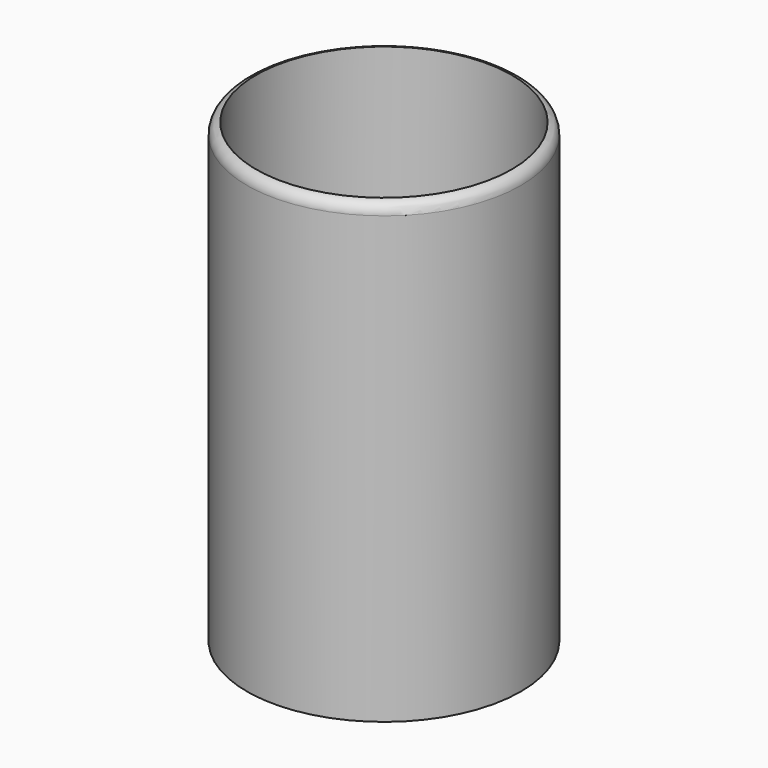
from build123d import *

# Parameters (mm, degrees)
F0_R     = 38.1
F1_DEPTH = 127
F2_T     = -2.54


# Not quite as in the source:
# - a fillet or chamfer that OpenCascade refuses, or shapes differently, is made with other operations: its cross-section is extruded or revolved along the edge and cut away or added


with BuildPart() as f1:
    # F0 (on Top) → F1 (new body)
    with BuildSketch(Plane.XY):
        Circle(F0_R)
    extrude(amount=F1_DEPTH)

    # F2
    f2_openings = [f1.faces().sort_by_distance(p)[0] for p in [
        (0, 0, 127),
    ]]
    offset(amount=F2_T, openings=f2_openings)

    # F3: fillet of radius 3.175 on 1 edges, made by hand

    # F3_s1 → F3_t2 (revolve, cut)
    with BuildSketch(Plane.XZ):
        with BuildLine():
            ThreePointArc((38.1, 123.8891480267), (37.3843444248, 125.8971943409), (35.56, 127))
            Line((35.56, 127), (38.1, 127))
            Line((38.1, 127), (38.1, 123.8891480267))
        make_face()
    revolve(axis=Axis((0, 0, 127), (0, 0, 1)), mode=Mode.SUBTRACT)


solid = f1.part
